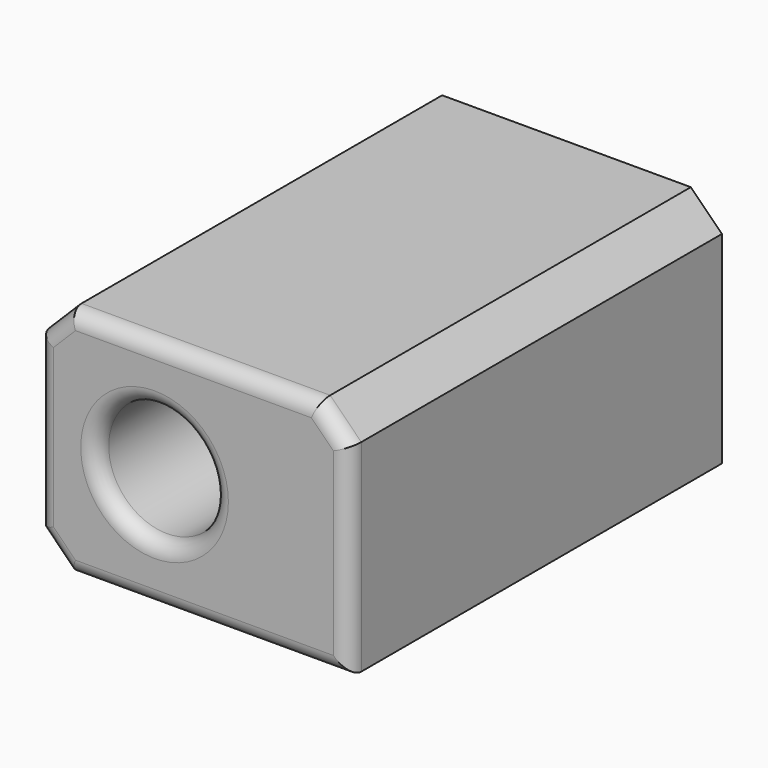
from build123d import *

# Parameters (mm, degrees)
F0_W     = 50.8
F0_H     = 38.1
F0_R     = 9.525
F1_DEPTH = 76.2
F2_SIZE  = 5.08
F3_SIZE  = 5.08
F4_R     = 2.54
F5_T     = 2.54


# Not quite as in the source:
# - a shell that OpenCascade refuses in one call is made with other operations: the cavity is built on its own and cut out


with BuildPart() as f1:
    # F0 (on Front) → F1 (new body)
    with BuildSketch(Plane.XZ):
        with Locations((25.4, 19.05)):
            Rectangle(F0_W, F0_H)
        with Locations((19.05, 19.05)):
            Circle(F0_R, mode=Mode.SUBTRACT)
    extrude(amount=F1_DEPTH)

    # F2
    f2_edges = [f1.edges().sort_by_distance(p)[0] for p in [
        (0, -38.1, 0),
    ]]
    chamfer(f2_edges, length=F2_SIZE)

    # F3
    f3_edges = [f1.edges().sort_by_distance(p)[0] for p in [
        (0, -38.1, 38.1),
        (50.8, -38.1, 38.1),
    ]]
    chamfer(f3_edges, length=F3_SIZE)

    # F4
    f4_edges = [f1.edges().sort_by_distance(p)[0] for p in [
        (0, -76.2, 19.05),
        (2.54, -76.2, 35.56),
        (2.54, -76.2, 2.54),
        (25.4, -76.2, 38.1),
        (27.94, -76.2, 0),
        (48.26, -76.2, 35.56),
        (50.8, -76.2, 16.51),
        (9.525, -76.2, 19.05),
    ]]
    fillet(f4_edges, radius=F4_R)

    # F5: shell of thickness 2.54, made by hand


with BuildPart() as f5_core1:
    # F5_t2: copy of F1
    add(f1.part)

    # the walls: a layer under each face that stays
    f5_faces = [f5_core1.faces().sort_by_distance(p)[0] for p in [
        (0, -36.83, 19.05),
        (2.54, -36.83, 35.56),
        (2.54, -36.83, 2.54),
        (25.4, -36.83, 38.1),
        (10.16, -76.2, 8.0433333333),
        (27.94, -36.83, 0),
        (48.26, -36.83, 35.56),
        (50.8, -36.83, 16.51),
        (9.525, -36.83, 19.05),
    ]]
    thicken(f5_faces, amount=-F5_T, mode=Mode.SUBTRACT)


with BuildPart() as f1_1:
    add(f1.part)

    # what is left inside the walls is the cavity
    f5_cavity = [f5_core1.part.solids().sort_by_distance(p)[0] for p in [
        (6.9596, -49.106667, 19.05),
    ]]
    add(f5_cavity, mode=Mode.SUBTRACT)


solid = f1_1.part
